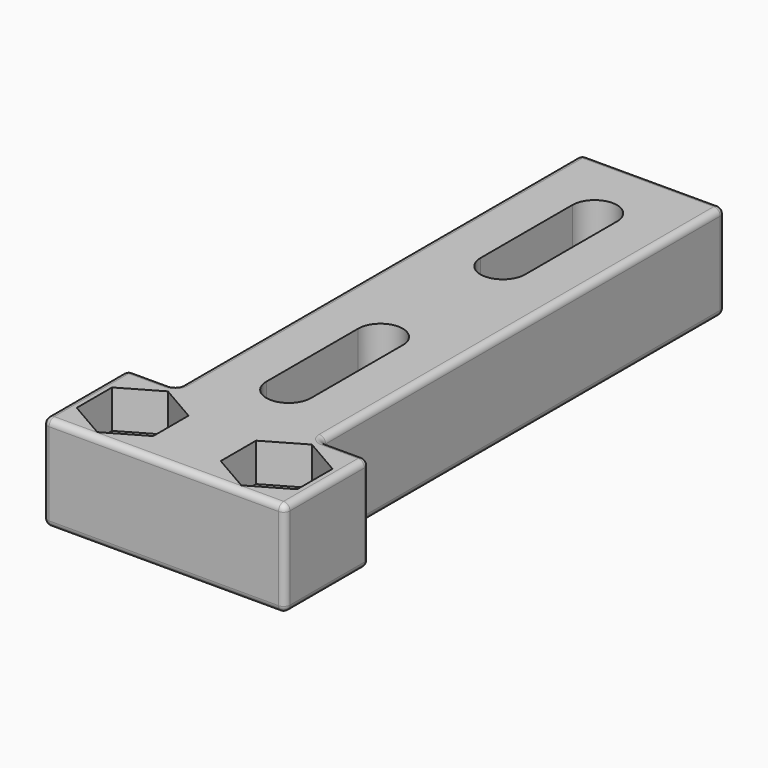
from build123d import *

# Parameters (mm, degrees)
F0_R     = 1.75
F1_DEPTH = 7.5
F2_DEPTH = 4.5
F3_DEPTH = 4.5
F5_DEPTH = 8.81
F7_DEPTH = 25
F8_F1_R  = 0.5
F8_F2_R  = 0.5


with BuildPart() as f1:
    # F0 (on Top) → F1 (new body)
    with BuildSketch(Plane.XY):
        Polygon((-9.5, 0), (-5.65, 0), (5.65, 0), (9.5, 0), (9.5, 8.3), (5.65, 8.3), (5.65, 10.5504491955), (5.65, 11.4643116325), (5.65, 48), (-5.65, 48), (-5.65, 8.3), (-9.5, 8.3), align=None)
        Polygon((-5.65, 7.4641016151), (-2.65, 5.7320508076), (-2.65, 2.2679491924), (-5.65, 0.5358983849), (-8.65, 2.2679491924), (-8.65, 5.7320508076), align=None, mode=Mode.SUBTRACT)
        Polygon((2.65, 5.7320508076), (5.65, 7.4641016151), (8.65, 5.7320508076), (8.65, 2.2679491924), (5.65, 0.5358983849), (2.65, 2.2679491924), align=None, mode=Mode.SUBTRACT)
        with Locations((0, 12.25)):
            Circle(F0_R, mode=Mode.SUBTRACT)
        with BuildLine():
            ThreePointArc((-1.7499927683, 21.255030998), (0.0025155016, 22.9999981921), (1.75, 21.25))
            ThreePointArc((1.75, 21.25), (1.7499981921, 21.2474844984), (1.7499927683, 21.244969002))
            ThreePointArc((1.7499927683, 21.244969002), (-0.005030998, 19.5000072317), (-1.7499927683, 21.255030998))
        make_face(mode=Mode.SUBTRACT)
        with BuildLine():
            ThreePointArc((-1.7499927683, 33.244969002), (-0.005030998, 34.9999927683), (1.7499927683, 33.255030998))
            ThreePointArc((1.7499927683, 33.255030998), (1.7499981921, 33.2525155016), (1.75, 33.25))
            ThreePointArc((1.75, 33.25), (0.0025155016, 31.5000018079), (-1.7499927683, 33.244969002))
        make_face(mode=Mode.SUBTRACT)
        with Locations((0, 42.25)):
            Circle(F0_R, mode=Mode.SUBTRACT)
    extrude(amount=F1_DEPTH)

    # F0 (on Top) → F2 (join)
    with BuildSketch(Plane.XY):
        Polygon((-2.65, 2.2679491924), (-2.65, 5.7320508076), (-5.65, 7.4641016151), (-8.65, 5.7320508076), (-8.65, 2.2679491924), (-5.65, 0.5358983849), align=None)
        with Locations((-5.65, 4)):
            Circle(F0_R, mode=Mode.SUBTRACT)
    extrude(amount=F2_DEPTH)

    # F0 (on Top) → F3 (join)
    with BuildSketch(Plane.XY):
        Polygon((8.65, 5.7320508076), (5.65, 7.4641016151), (2.65, 5.7320508076), (2.65, 2.2679491924), (5.65, 0.5358983849), (8.65, 2.2679491924), align=None)
        with Locations((5.65, 4)):
            Circle(F0_R, mode=Mode.SUBTRACT)
    extrude(amount=F3_DEPTH)

    # F4 (on face) → F5 (cut)
    with BuildSketch(Plane.XY.offset(7.5)):
        with BuildLine():
            Line((-1.75, 21.25), (-1.75, 12.25))
            ThreePointArc((-1.75, 12.25), (0, 14), (1.75, 12.25))
            Line((1.75, 12.25), (1.75, 21.25))
            ThreePointArc((1.75, 21.25), (0, 19.5), (-1.75, 21.25))
        make_face()
    extrude(amount=-F5_DEPTH, mode=Mode.SUBTRACT)

    # F6 (on face) → F7 (cut)
    with BuildSketch(Plane.XY.offset(7.5)):
        with BuildLine():
            Line((-1.75, 42.25), (-1.75, 33.25))
            ThreePointArc((-1.75, 33.25), (0, 35), (1.75, 33.25))
            Line((1.75, 33.25), (1.75, 42.25))
            ThreePointArc((1.75, 42.25), (0, 40.5), (-1.75, 42.25))
        make_face()
    extrude(amount=-F7_DEPTH, mode=Mode.SUBTRACT)

    # F8: fillet of radius 0.5 on 20 edges, made by hand

    # F8_f1
    f8_f1_edges = [f1.edges().sort_by_distance(p)[0] for p in [
        (5.65, 8.3, 3.75),
        (-5.65, 8.3, 3.75),
    ]]
    fillet(f8_f1_edges, radius=F8_F1_R)

    # F8_f2
    f8_f2_edges = [f1.edges().sort_by_distance(p)[0] for p in [
        (-5.65, 48, 3.75),
        (5.65, 48, 3.75),
        (9.5, 8.3, 3.75),
        (-9.5, 8.3, 3.75),
        (-9.5, 0, 3.75),
        (9.5, 0, 3.75),
        (9.5, 4.15, 0),
        (9.5, 4.15, 7.5),
        (5.65, 28.4, 7.5),
        (5.65, 28.4, 0),
        (-5.65, 28.4, 0),
        (-5.65, 28.4, 7.5),
        (-9.5, 4.15, 0),
        (-9.5, 4.15, 7.5),
        (0, 48, 0),
        (0, 48, 7.5),
        (0, 0, 7.5),
        (0, 0, 0),
        (-5.7964466094, 8.4464466094, 7.5),
        (-5.7964466094, 8.4464466094, 0),
        (5.7964466094, 8.4464466094, 0),
        (5.7964466094, 8.4464466094, 7.5),
    ]]
    fillet(f8_f2_edges, radius=F8_F2_R)


solid = f1.part
